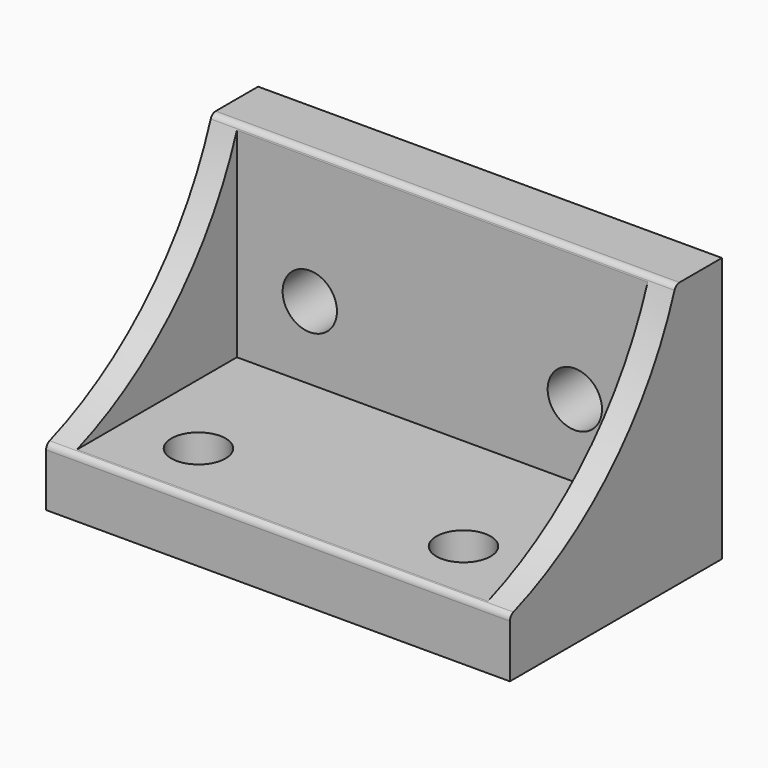
from build123d import *

# Parameters (mm, degrees)
F1_DEPTH = 35
F2_R     = 4.1
F3_DEPTH = 31
F4_DEPTH = 40.001
F5_R     = 4.1
F6_DEPTH = 19.2509998957


# Not quite as in the source:
# - ends of sketch curves that miss each other by under 0.0002 mm in the source are joined


with BuildPart() as f1:
    # F0 (on Right) → F1 (new body, symmetric)
    with BuildSketch(Plane.YZ):
        with BuildLine():
            ThreePointArc((0.6654529791, -10.3075948367), (0.1831243905, -10.6731600274), (3e-10, -11.2499998957))
            Line((3e-10, -11.2499998957), (0, -19.2499998957))
            Line((0, -19.2499998957), (40, -19.2499998957))
            Line((40, -19.2499998957), (40, 20.7500001043))
            Line((40, 20.7500001043), (32, 20.7500001043))
            ThreePointArc((32, 20.7500001043), (31.4231601317, 20.5668757138), (31.057594941, 20.0845471252))
            ThreePointArc((31.057594941, 20.0845471252), (19.2938390593, 1.456161045), (0.6654529791, -10.3075948367))
        make_face()
    extrude(amount=F1_DEPTH, both=True)

    # F2 (on Front) → F3 (cut)
    with BuildSketch(Plane.XZ):
        Polygon((-15.9000523031, -10.2499328405), (15.8999476969, -10.2499328405), (19.9999476969, -10.2499328405), (24.0999476969, -10.2499328405), (30.9999476969, -10.2499328405), (30.9999476969, 19.9232501595), (-31.0000523031, 19.9232501595), (-31.0000523031, -10.2499328405), (-24.1000523031, -10.2499328405), (-20.0000523031, -10.2499328405), align=None)
        with Locations((-20.0000523031, 0.7500671595)):
            Circle(F2_R, mode=Mode.SUBTRACT)
        with Locations((19.9999476969, 0.7500671595)):
            Circle(F2_R, mode=Mode.SUBTRACT)
        with Locations((-20.0000523031, 0.7500671595)):
            Circle(F2_R)
        with Locations((19.9999476969, 0.7500671595)):
            Circle(F2_R)
    extrude(amount=-F3_DEPTH, mode=Mode.SUBTRACT)

    # F2 (on Front) → F4 (cut, through all)
    with BuildSketch(Plane.XZ):
        with Locations((19.9999476969, 0.7500671595)):
            Circle(F2_R)
        with Locations((-20.0000523031, 0.7500671595)):
            Circle(F2_R)
    extrude(amount=-F4_DEPTH, mode=Mode.SUBTRACT)

    # F5 (on Top) → F6 (cut, through all)
    with BuildSketch(Plane.XY):
        with Locations((-20.000027626, 10)):
            Circle(F5_R)
        with Locations((19.999972374, 10)):
            Circle(F5_R)
    extrude(amount=-F6_DEPTH, mode=Mode.SUBTRACT)


solid = f1.part
